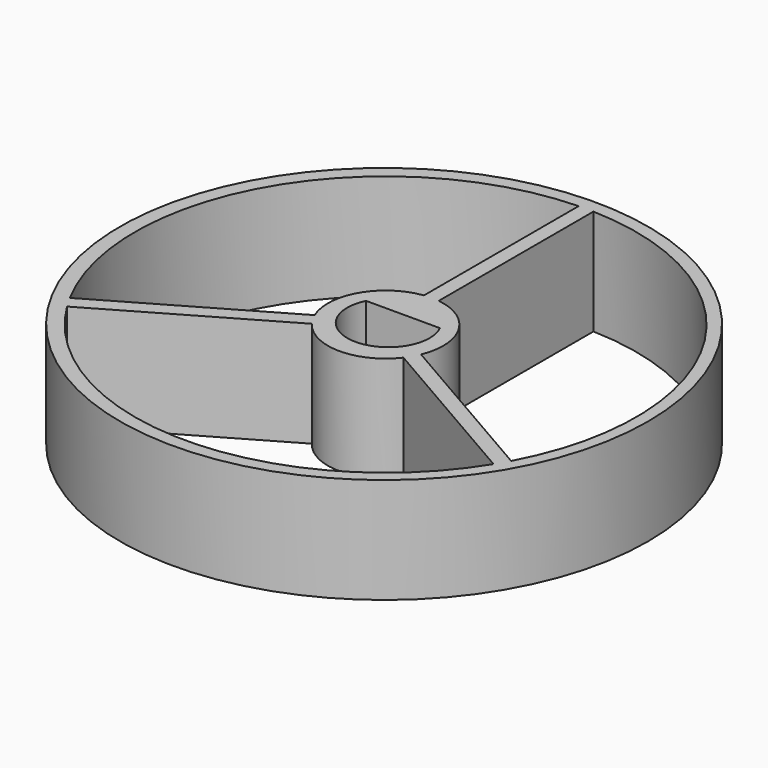
from build123d import *

# Parameters (mm, degrees)
F0_R     = 25
F1_DEPTH = 10


# Not quite as in the source:
# - a feature names something its author has since deleted; it is built from what else it names


with BuildPart() as f1:
    # F0 (on Top) → F1 (new body)
    with BuildSketch(Plane.XY):
        with Locations((-0.1409200142, -0.0023476887)):
            Circle(F0_R)
        with BuildLine():
            ThreePointArc((0.7, 23.7306175986), (17.033068856, 16.5380402997), (23.7409395688, 0))
            ThreePointArc((23.7409395688, 0), (23.0200904836, -5.8058286004), (20.9013176879, -11.2590910166))
            ThreePointArc((20.9013176879, -11.2590910166), (20.5602567763, -11.8704697844), (20.2013176879, -12.4715265819))
            ThreePointArc((20.2013176879, -12.4715265819), (0, -23.7409395688), (-20.2013176879, -12.4715265819))
            ThreePointArc((-20.2013176879, -12.4715265819), (-20.5602567763, -11.8704697844), (-20.9013176879, -11.2590910166))
            ThreePointArc((-20.9013176879, -11.2590910166), (-20.5602567763, 11.8704697844), (-0.7, 23.7306175986))
            ThreePointArc((-0.7, 23.7306175986), (0, 23.7409395688), (0.7, 23.7306175986))
        make_face(mode=Mode.SUBTRACT)
        with BuildLine():
            ThreePointArc((5.4607696164, 0), (4.1013743754, 3.6053755749), (0.7, 5.4157183091))
            ThreePointArc((0.7, 5.4157183091), (0.3507241153, 5.4494951508), (0, 5.4607696164))
            ThreePointArc((0, 5.4607696164), (-0.3507241153, 5.4494951508), (-0.7, 5.4157183091))
            ThreePointArc((-0.7, 5.4157183091), (-4.729165212, 2.7303848082), (-5.0401496354, -2.1016413719))
            ThreePointArc((-5.0401496354, -2.1016413719), (-4.8947632961, -2.4210115818), (-4.729165212, -2.7303848082))
            ThreePointArc((-4.729165212, -2.7303848082), (-4.5440391807, -3.028483569), (-4.3401496354, -3.3140769372))
            ThreePointArc((-4.3401496354, -3.3140769372), (0, -5.4607696164), (4.3401496354, -3.3140769372))
            ThreePointArc((4.3401496354, -3.3140769372), (4.5440391807, -3.028483569), (4.729165212, -2.7303848082))
            ThreePointArc((4.729165212, -2.7303848082), (4.8947632961, -2.4210115818), (5.0401496354, -2.1016413719))
            ThreePointArc((5.0401496354, -2.1016413719), (5.354582187, -1.0716596503), (5.4607696164, 0))
        make_face()
        with BuildLine():
            Line((-3.4987264855, 2.0612527399), (0, 2.0612527399))
            Line((0, 2.0612527399), (3.4987264855, 2.0612527399))
            ThreePointArc((3.4987264855, 2.0612527399), (0, -3.5618006487), (-3.4987264855, 2.0612527399))
        make_face(mode=Mode.SUBTRACT)
        with BuildLine():
            Line((-5.0401496354, -2.1016413719), (-20.9013176879, -11.2590910166))
            ThreePointArc((-20.9013176879, -11.2590910166), (-20.5602567763, -11.8704697844), (-20.2013176879, -12.4715265819))
            Line((-20.2013176879, -12.4715265819), (-4.3401496354, -3.3140769372))
            ThreePointArc((-4.3401496354, -3.3140769372), (-4.5440391807, -3.028483569), (-4.729165212, -2.7303848082))
            ThreePointArc((-4.729165212, -2.7303848082), (-4.8947632961, -2.4210115818), (-5.0401496354, -2.1016413719))
        make_face()
        with BuildLine():
            Line((0.7, 5.4157183091), (0.7, 23.7306175986))
            ThreePointArc((0.7, 23.7306175986), (0, 23.7409395688), (-0.7, 23.7306175986))
            Line((-0.7, 23.7306175986), (-0.7, 5.4157183091))
            ThreePointArc((-0.7, 5.4157183091), (-0.3507241153, 5.4494951508), (0, 5.4607696164))
            ThreePointArc((0, 5.4607696164), (0.3507241153, 5.4494951508), (0.7, 5.4157183091))
        make_face()
        with BuildLine():
            ThreePointArc((20.2013176879, -12.4715265819), (20.5602567763, -11.8704697844), (20.9013176879, -11.2590910166))
            Line((20.9013176879, -11.2590910166), (5.0401496354, -2.1016413719))
            ThreePointArc((5.0401496354, -2.1016413719), (4.8947632961, -2.4210115818), (4.729165212, -2.7303848082))
            ThreePointArc((4.729165212, -2.7303848082), (4.5440391807, -3.028483569), (4.3401496354, -3.3140769372))
            Line((4.3401496354, -3.3140769372), (20.2013176879, -12.4715265819))
        make_face()
    extrude(amount=F1_DEPTH)


solid = f1.part
